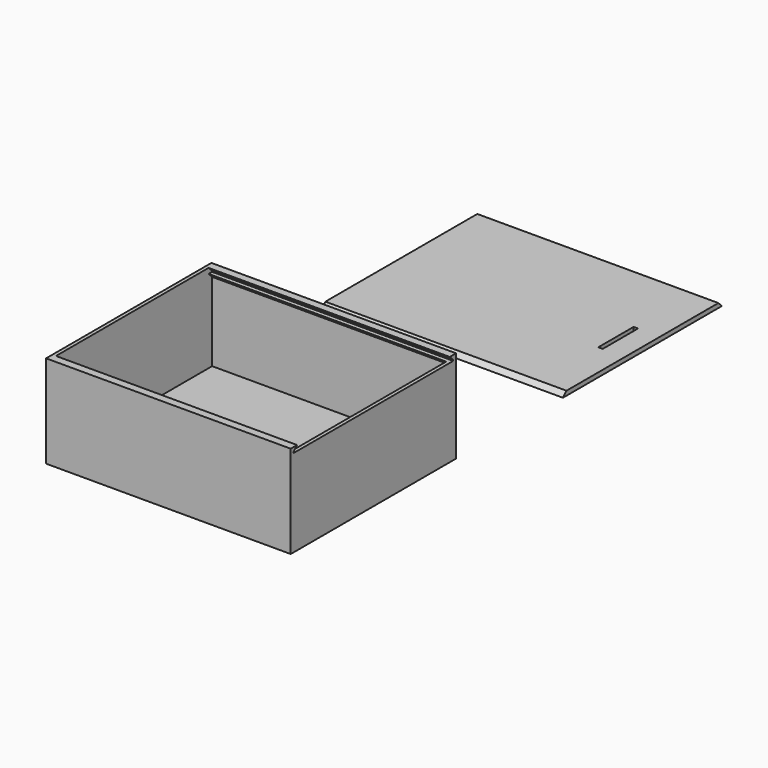
from build123d import *

# Parameters (mm, degrees)
F0_W       = 55.4
F0_H       = 46.8
F0_W_2     = 53.8
F0_H_2     = 45.2
F1_DEPTH   = 21
F2_DEPTH   = 1
F3_W       = 53.8
F3_H       = 1
F5_DEPTH   = 1
F4_W       = 53.8
F4_H       = 1
F6_DEPTH   = 1
F9_DEPTH   = 0.8
F0_W_3     = 54.6
F0_H_3     = 45
F0_W_4     = 1
F0_H_4     = 10
F10_DEPTH  = 1
F11_SIZE   = 0.99999
F11_2_SIZE = 0.99999


# Not quite as in the source:
# - a fillet or chamfer is up to 0.001 mm smaller than in the source, because OpenCascade refuses the exact size
# - a feature of the source that left no trace in its solid (it failed there, or was rolled back) is left out
# - a feature names something its author has since deleted; it is built from what else it names


with BuildPart() as f1:
    # F0 (on Top) → F1 (new body)
    with BuildSketch(Plane.XY):
        with Locations((26.9, -22.6)):
            Rectangle(F0_W, F0_H)
        with Locations((26.9, -22.6)):
            Rectangle(F0_W_2, F0_H_2, mode=Mode.SUBTRACT)
    extrude(amount=F1_DEPTH)

    # F0 (on Top) → F2 (join)
    with BuildSketch(Plane.XY):
        with Locations((26.9, -22.6)):
            Rectangle(F0_W_2, F0_H_2)
    extrude(amount=F2_DEPTH)

    # F3 (on face) → F5 (join)
    with BuildSketch(Plane(origin=(0, -45.2, 0), x_dir=(-1, 0, 0), z_dir=(0, 1, 0))):
        with Locations((-26.9, 20.5)):
            Rectangle(F3_W, F3_H)
        with Locations((-26.9, 19.3)):
            Rectangle(F3_W, F3_H)
    extrude(amount=F5_DEPTH)

    # F4 (on face) → F6 (join)
    with BuildSketch(Plane.XZ):
        with Locations((26.9, 19.3)):
            Rectangle(F4_W, F4_H)
        with Locations((26.9, 20.5)):
            Rectangle(F4_W, F4_H)
    extrude(amount=F6_DEPTH)

    # F8 (on face) → F9 (cut, through all)
    with BuildSketch(Plane(origin=(53.8, 0, 0), x_dir=(0, -1, 0), z_dir=(-1, 0, 0))):
        Polygon((0, 19.8), (1, 19.8), (44.2, 19.8), (45.2, 19.8), (45.2, 20), (44.2, 20), (44.2, 21), (1, 21), (1, 20), (0, 20), align=None)
    extrude(amount=-F9_DEPTH, mode=Mode.SUBTRACT)

    # F11#2 (size 1 in the source; OpenCascade refuses exactly that, so slightly less here)
    f11_2_edges = [f1.edges().sort_by_distance(p)[0] for p in [
        (27.3, -1, 20),
        (26.9, -1, 18.8),
        (26.9, -44.2, 18.8),
        (27.3, -44.2, 20),
    ]]
    chamfer(f11_2_edges, length=F11_2_SIZE)


with BuildPart() as f10:
    # F0 (on Top) → F10 (new body)
    with BuildSketch(Plane.XY):
        with Locations((27.5, 53.3)):
            Rectangle(F0_W_3, F0_H_3)
        with Locations((49.3, 53.3)):
            Rectangle(F0_W_4, F0_H_4, mode=Mode.SUBTRACT)
    extrude(amount=F10_DEPTH)

    # F11 (size 1 in the source; OpenCascade refuses exactly that, so slightly less here)
    f11_edges = [f10.edges().sort_by_distance(p)[0] for p in [
        (27.5, 30.8, 1),
        (27.5, 75.8, 1),
    ]]
    chamfer(f11_edges, length=F11_SIZE)


solid = Compound([f1.part, f10.part])
